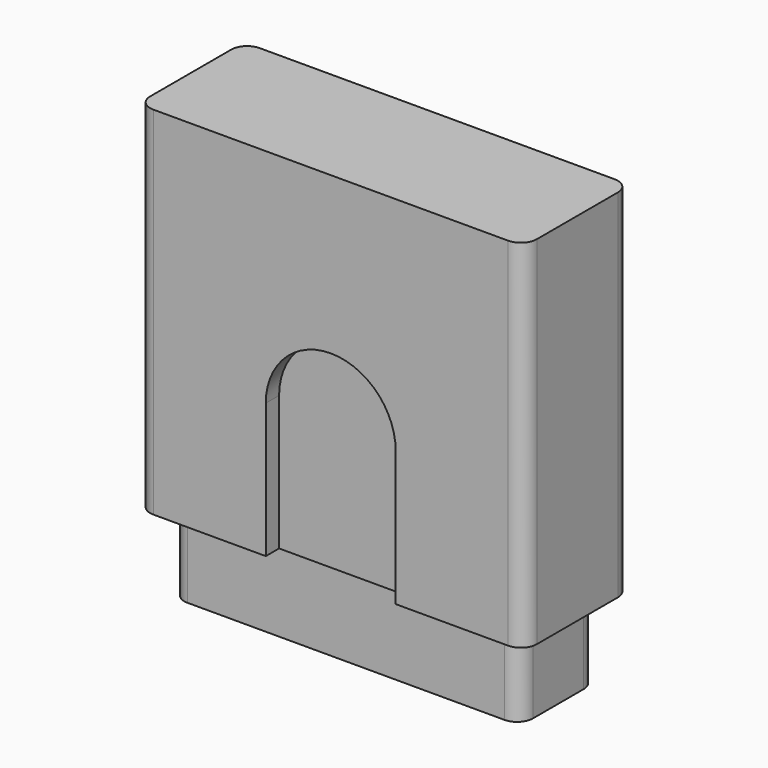
from build123d import *

# Parameters (mm, degrees)
F0_W     = 48.799998641
F0_H     = 16.799998641
F0_W_2   = 44.799998641
F0_H_2   = 12.799998641
F0_W_3   = 44
F0_H_3   = 12
F0_W_4   = 40
F0_H_4   = 8
F1_DEPTH = 45
F2_DEPTH = 42
F3_DEPTH = 10
F4_R     = 2
F5_R     = 2
F6_R     = 2
F8_DEPTH = 25.2
F9_R     = 8.19999


# Not quite as in the source:
# - a fillet or chamfer is up to 0.001 mm smaller than in the source, because OpenCascade refuses the exact size


with BuildPart() as f1:
    # F0 (on Top) → F1 (new body)
    with BuildSketch(Plane.XY):
        with Locations((-3.2957775742, 1.1005828176)):
            Rectangle(F0_W, F0_H)
        with Locations((-3.2957775742, 1.1005828176)):
            Rectangle(F0_W_2, F0_H_2, mode=Mode.SUBTRACT)
        with Locations((-3.2957775742, 1.1005828176)):
            Rectangle(F0_W_2, F0_H_2)
        with Locations((-3.2957775742, 1.1005828176)):
            Rectangle(F0_W_3, F0_H_3, mode=Mode.SUBTRACT)
        with Locations((-3.2957775742, 1.1005828176)):
            Rectangle(F0_W_3, F0_H_3)
        with Locations((-3.2957775742, 1.1005828176)):
            Rectangle(F0_W_4, F0_H_4, mode=Mode.SUBTRACT)
        with Locations((-3.2957775742, 1.1005828176)):
            Rectangle(F0_W_4, F0_H_4)
    extrude(amount=F1_DEPTH)

    # F0 (on Top) → F2 (cut)
    with BuildSketch(Plane.XY):
        with Locations((-3.2957775742, 1.1005828176)):
            Rectangle(F0_W_4, F0_H_4)
    extrude(amount=F2_DEPTH, mode=Mode.SUBTRACT)

    # F0 (on Top) → F3 (join)
    with BuildSketch(Plane.XY):
        with Locations((-3.2957775742, 1.1005828176)):
            Rectangle(F0_W_3, F0_H_3)
        with Locations((-3.2957775742, 1.1005828176)):
            Rectangle(F0_W_4, F0_H_4, mode=Mode.SUBTRACT)
    extrude(amount=-F3_DEPTH)

    # F4
    f4_edges = [f1.edges().sort_by_distance(p)[0] for p in [
        (-27.695777, -7.299417, 22.5),
        (-27.695777, 9.500582, 22.5),
        (21.104222, -7.299417, 22.5),
        (21.104222, 9.500582, 22.5),
    ]]
    fillet(f4_edges, radius=F4_R)

    # F5
    f5_edges = [f1.edges().sort_by_distance(p)[0] for p in [
        (-23.295778, 5.100583, 16),
        (-23.295778, -2.899417, 16),
        (16.704222, 5.100583, 16),
        (16.704222, -2.899417, 16),
    ]]
    fillet(f5_edges, radius=F5_R)

    # F6
    f6_edges = [f1.edges().sort_by_distance(p)[0] for p in [
        (18.704222, -4.899417, -5),
        (18.704222, 7.100583, -5),
        (-25.295778, -4.899417, -5),
        (-25.295778, 7.100583, -5),
    ]]
    fillet(f6_edges, radius=F6_R)

    # F7 (on face) → F8 (cut)
    with BuildSketch(Plane(origin=(0, 0, 0), x_dir=(1, 0, 0), z_dir=(0, 0, -1))):
        Polygon((4.9042224258, 7.2994165029), (-3.2957775742, 7.2994165029), (-11.4957775742, 7.2994165029), (-11.4957775742, 5.1994165029), (4.9042224258, 5.1994165029), align=None)
        Polygon((-3.2957775742, -9.5005821381), (4.9042224258, -9.5005821381), (4.9042224258, -7.4005821381), (-11.4957775742, -7.4005821381), (-11.4957775742, -9.5005821381), align=None)
    extrude(amount=-F8_DEPTH, mode=Mode.SUBTRACT)

    # F9 (radius 8.2 in the source; OpenCascade refuses exactly that, so slightly less here)
    f9_edges = [f1.edges().sort_by_distance(p)[0] for p in [
        (-11.495778, -6.249417, 25.2),
        (4.904222, -6.249417, 25.2),
        (4.904222, 8.450582, 25.2),
        (-11.495778, 8.450582, 25.2),
    ]]
    fillet(f9_edges, radius=F9_R)


solid = f1.part
